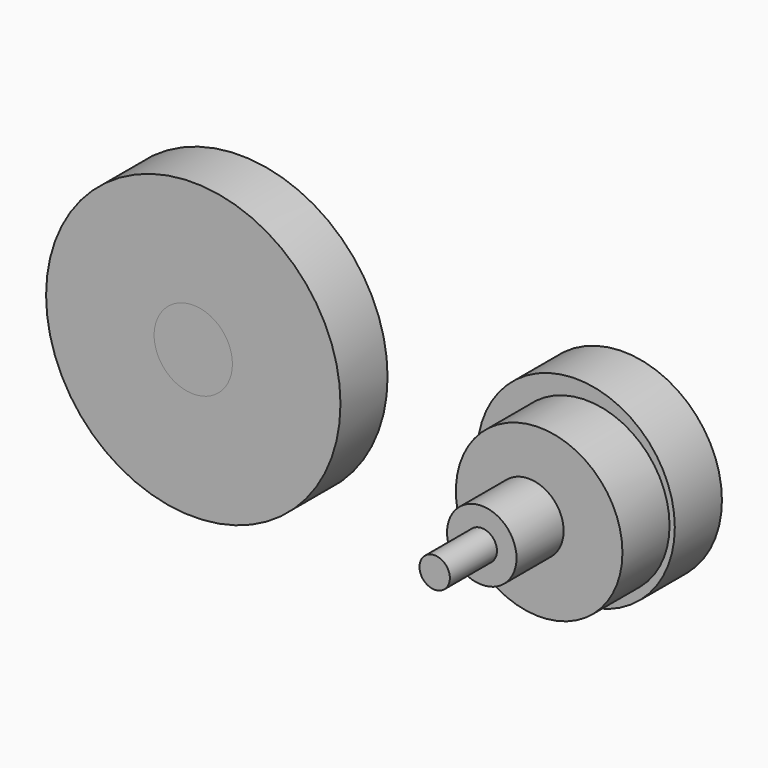
from build123d import *

# Parameters (mm, degrees)
F0_R     = 42.6433885457
F2_DEPTH = 25.4
F0_R_2   = 63.5
F1_R     = 63.5
F1_R_2   = 16.8845262582
F3_R     = 35.9345767258
F3_R_2   = 14.9934405288
F4_DEPTH = 25.4
F5_DEPTH = 50.8
F6_R     = 6.5529414014
F7_DEPTH = 25.4


with BuildPart() as f2:
    # F0 (on Front) → F2 (new body)
    with BuildSketch(Plane.XZ):
        with Locations((165.1, 0)):
            Circle(F0_R)
    extrude(amount=F2_DEPTH)

    # F3 (on face) → F4 (join)
    with BuildSketch(Plane.XZ.offset(25.4)):
        with Locations((169.5338785648, 0)):
            Circle(F3_R)
        with Locations((165.1, 0)):
            Circle(F3_R_2, mode=Mode.SUBTRACT)
    extrude(amount=F4_DEPTH)

    # F5 (add): a face of the model
    f5_faces = [f2.faces().sort_by_distance(p)[0] for p in [
        (165.1, -25.4, 0),
    ]]
    extrude(f5_faces, amount=F5_DEPTH)

    # F6 (on face) → F7 (join)
    with BuildSketch(Plane.XZ.offset(76.2)):
        with Locations((165.1, 0)):
            Circle(F6_R)
    extrude(amount=F7_DEPTH)


with BuildPart() as f2b:
    # F0 (on Front) → F2, piece 2 (new body)
    with BuildSketch(Plane.XZ):
        Circle(F0_R_2)
    extrude(amount=F2_DEPTH)


with BuildPart() as f2c:
    # F1 (on face) → F2, piece 3 (new body)
    with BuildSketch(Plane.XZ):
        Circle(F1_R)
        Circle(F1_R_2, mode=Mode.SUBTRACT)
    extrude(amount=F2_DEPTH)


solid = Compound([f2.part, f2b.part, f2c.part])
